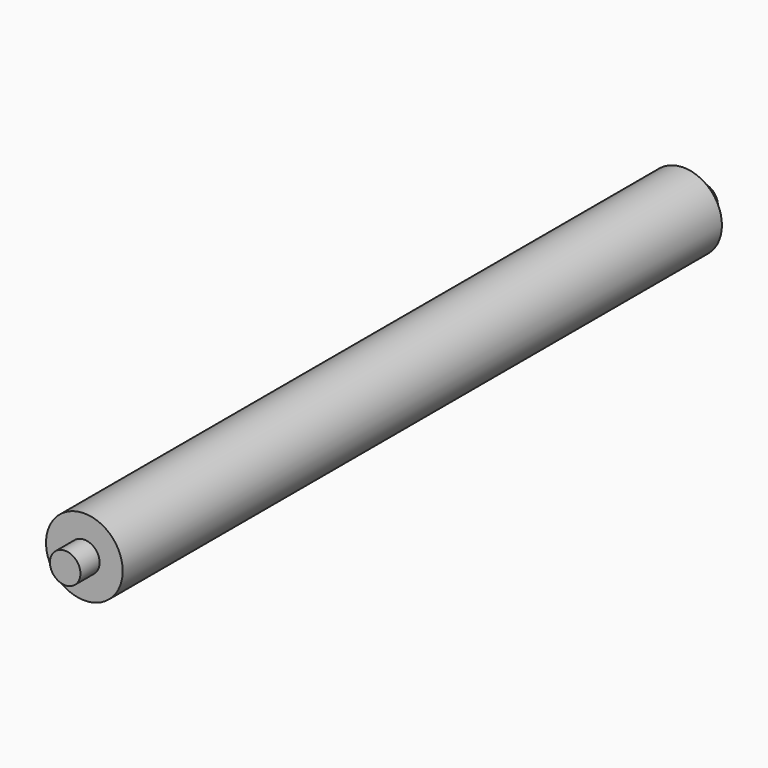
from build123d import *

# Parameters (mm, degrees)
F0_R     = 8
F1_DEPTH = 156.25
F2_R     = 3.175
F3_DEPTH = 5


# Not quite as in the source:
# - a pattern or mirror of a feature is missing from the dataset's text; its kind, count and spacing are read off the source's solid


with BuildPart() as f1:
    # F0 (on Front) → F1 (new body)
    with BuildSketch(Plane.XZ):
        Circle(F0_R)
    extrude(amount=F1_DEPTH)


with BuildPart() as f3:
    # F2 (on face) → F3 (new body)
    with BuildSketch(Plane.XZ.offset(156.25)):
        Circle(F2_R)
    extrude(amount=F3_DEPTH)


with BuildPart() as f3_copies_1:
    # F3_copies: instance of F3
    add(f3.part.mirror(Plane.ZX.offset(-78.125)))


solid = Compound([f1.part, f3.part, f3_copies_1.part])
